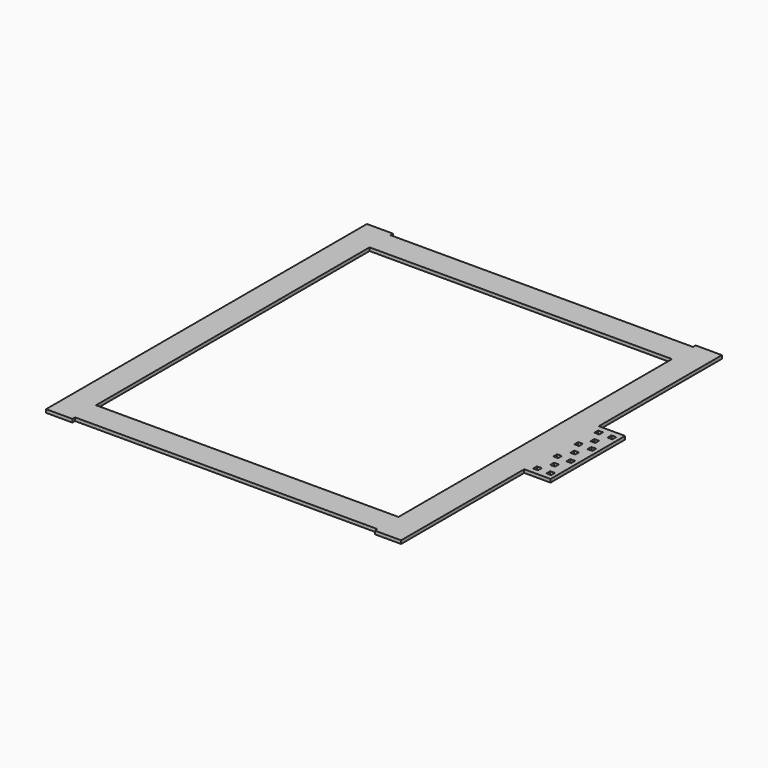
from build123d import *

# Parameters (mm, degrees)
F0_W     = 4.6228
F0_H     = 4.6228
F0_W_2   = 292.1
F0_H_2   = 330.2
F1_DEPTH = 3.175


# Not quite as in the source:
# - a length typed as a fraction of an inch, garbled in the dataset ("3 / 203.2 mm" for 3/8 in), is restored


with BuildPart() as f1:
    # F0 (on Top) → F1 (new body)
    with BuildSketch(Plane.XY):
        Polygon((190.4998123646, 755.6496634722), (190.4998123646, 635.6350152016), (190.4998123646, 610.2350152016), (190.4998123646, 607.0600152016), (215.8998123646, 607.0600152016), (215.8998123646, 610.2350152016), (507.9998123646, 610.2350152016), (507.9998123646, 607.0600152016), (533.3998123646, 607.0600152016), (533.3998123646, 610.2350152016), (533.3998123646, 755.7291580558), (558.7998123646, 755.7291580558), (558.7998123646, 760.8061958763), (558.7998123646, 800.7350152016), (558.7998123646, 845.7408688016), (533.3998123646, 845.7408688016), (533.3998123646, 991.2350152016), (533.3998123646, 994.4100152016), (507.9998123646, 994.4100152016), (507.9998123646, 991.2350152016), (215.8998123646, 991.2350152016), (215.8998123646, 994.4100152016), (190.4998123646, 994.4100152016), (190.4998123646, 991.2350152016), (190.4998123646, 857.2496634722), align=None)
        with Locations((540.2533960062, 763.1175958763)):
            Rectangle(F0_W, F0_H, mode=Mode.SUBTRACT)
        with Locations((552.9533960062, 763.1175958763)):
            Rectangle(F0_W, F0_H, mode=Mode.SUBTRACT)
        with Locations((546.5928981277, 775.8096898529)):
            Rectangle(F0_W, F0_H, mode=Mode.SUBTRACT)
        with Locations((539.7752002493, 788.0271025263)):
            Rectangle(F0_W, F0_H, mode=Mode.SUBTRACT)
        with Locations((552.4752002493, 788.0271025263)):
            Rectangle(F0_W, F0_H, mode=Mode.SUBTRACT)
        with Locations((546.1356981277, 800.7350085497)):
            Rectangle(F0_W, F0_H, mode=Mode.SUBTRACT)
        with Locations((361.9498123646, 800.7350152016)):
            Rectangle(F0_W_2, F0_H_2, mode=Mode.SUBTRACT)
        with Locations((539.7752002493, 813.4271025263)):
            Rectangle(F0_W, F0_H, mode=Mode.SUBTRACT)
        with Locations((552.4752002493, 813.4271025263)):
            Rectangle(F0_W, F0_H, mode=Mode.SUBTRACT)
        with Locations((546.1356981277, 824.9666085497)):
            Rectangle(F0_W, F0_H, mode=Mode.SUBTRACT)
        with Locations((539.7752002493, 837.6587025263)):
            Rectangle(F0_W, F0_H, mode=Mode.SUBTRACT)
        with Locations((552.4752002493, 837.6587025263)):
            Rectangle(F0_W, F0_H, mode=Mode.SUBTRACT)
    extrude(amount=F1_DEPTH)


solid = f1.part
